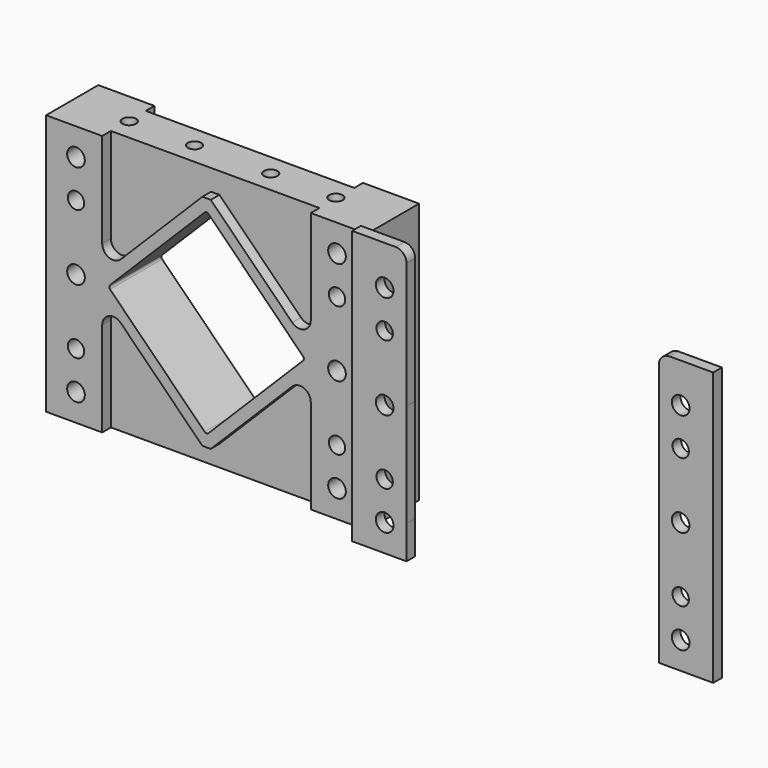
from build123d import *

# Parameters (mm, degrees)
F0_W      = 187.325
F0_H      = 152.4
F1_DEPTH  = 38.1
F3_D      = 9.5758
F4_DEPTH  = 6.35
F6_DEPTH  = 6.35
F8_D      = 7.9375
F8_DEPTH  = 22.225
F8_TIP    = 2.3846655818
F10_D     = 7.9375
F10_DEPTH = 22.225
F10_TIP   = 2.3846655818
F11_D     = 10.3124
F12_R     = 5.1562
F12_R_2   = 4.7879
F13_DEPTH = 6.35
F14_ANGLE = 180
F16_ANGLE = 180


# Not quite as in the source:
# - ends of sketch curves that miss each other by under 0.0002 mm in the source are joined


with BuildPart() as f1:
    # F0 (on Front) → F1 (new body)
    with BuildSketch(Plane.XZ):
        with Locations((17.3622183502, -12.1438738748)):
            Rectangle(F0_W, F0_H)
        with BuildLine():
            ThreePointArc((73.7470006338, -11.0550622269), (74.2119686187, -12.1775942421), (73.7470006338, -13.3001262572))
            Line((73.7470006338, -13.3001262572), (18.5184254892, -68.5287014018))
            ThreePointArc((18.5184254892, -68.5287014018), (17.3958934741, -68.9936693866), (16.273361459, -68.5287014018))
            Line((16.273361459, -68.5287014018), (-38.9552136856, -13.3001262572))
            ThreePointArc((-38.9552136856, -13.3001262572), (-39.4201816705, -12.1775942421), (-38.9552136856, -11.0550622269))
            Line((-38.9552136856, -11.0550622269), (16.273361459, 44.1735129177))
            ThreePointArc((16.273361459, 44.1735129177), (17.3958934741, 44.6384809025), (18.5184254892, 44.1735129177))
            Line((18.5184254892, 44.1735129177), (73.7470006338, -11.0550622269))
        make_face(mode=Mode.SUBTRACT)
    extrude(amount=F1_DEPTH)

    # F3 (through all)
    with Locations(Plane(origin=(0, 0, 0), x_dir=(1, 0, 0), z_dir=(0, 1, 0))):
        with Locations((-58.8377816498, -25.9561261252), (-58.8377816498, 50.2438738748), (93.5622183502, 50.2438738748), (93.5622183502, -25.9561261252)):
            Hole(F3_D / 2)

    # F2 (on face) → F4 (cut)
    with BuildSketch(Plane.XZ.offset(38.1)):
        with BuildLine():
            Line((-32.6721932196, 4.2082143602), (14.9574931524, 51.8379007322))
            Line((14.9574931524, 51.8379007322), (17.3622183502, 51.8379006441))
            Line((17.3622183502, 51.8379006441), (17.3622183502, 64.0561261252))
            Line((17.3622183502, 64.0561261252), (-43.5123212801, 64.0561261252))
            Line((-43.5123212801, 64.0561261252), (-43.5123212801, 8.6983424207))
            ThreePointArc((-43.5123212801, 8.6983424207), (-39.5923610756, 2.8317073892), (-32.6721932196, 4.2082143602))
        make_face()
        with BuildLine():
            Line((17.3622183502, 64.0561261252), (17.3622183502, 51.8379006441))
            Line((17.3622183502, 51.8379006441), (19.8342931524, 51.8379005536))
            Line((19.8342931524, 51.8379005536), (67.3966299199, 4.2755637861))
            ThreePointArc((67.3966299199, 4.2755637861), (74.316797776, 2.8990568152), (78.2367579805, 8.7656918466))
            Line((78.2367579805, 8.7656918466), (78.2367579805, 64.0561261252))
            Line((78.2367579805, 64.0561261252), (17.3622183502, 64.0561261252))
        make_face()
        with BuildLine():
            Line((19.8340516262, -76.1933300919), (17.3558846933, -76.1930850326))
            Line((17.3558846933, -76.1930850326), (17.354683134, -88.3438738748))
            Line((17.354683134, -88.3438738748), (78.2360174681, -88.3438738748))
            Line((78.2360174681, -88.3438738748), (78.2360174681, -33.1216203711))
            ThreePointArc((78.2360174681, -33.1216203711), (74.3160572637, -27.2549853396), (67.3958894076, -28.6314923106))
            Line((67.3958894076, -28.6314923106), (19.8340516262, -76.1933300919))
        make_face()
        with BuildLine():
            Line((17.354683134, -88.3438738748), (17.3558846933, -76.1930850326))
            Line((17.3558846933, -76.1930850326), (14.9572517743, -76.1928478381))
            Line((14.9572517743, -76.1928478381), (-32.6714527073, -28.5641433566))
            ThreePointArc((-32.6714527073, -28.5641433566), (-39.5916205633, -27.1876363857), (-43.5115807678, -33.0542714171))
            Line((-43.5115807678, -33.0542714171), (-43.5115807678, -88.3438738748))
            Line((-43.5115807678, -88.3438738748), (17.354683134, -88.3438738748))
        make_face()
    extrude(amount=-F4_DEPTH, mode=Mode.SUBTRACT)

    # F5 (on face) → F6 (cut)
    with BuildSketch(Plane.XZ):
        with BuildLine():
            Line((78.2333183502, -88.3438738748), (78.2333183502, -76.2026738748))
            Line((78.2333183502, -76.2026738748), (78.2333183502, -33.1243194891))
            ThreePointArc((78.2333183502, -33.1243194891), (74.3133581457, -27.2576844576), (67.3931902896, -28.6341914285))
            Line((67.3931902896, -28.6341914285), (19.8247078433, -76.2026738748))
            Line((19.8247078433, -76.2026738748), (14.967077811, -76.2026738748))
            Line((14.967077811, -76.2026738748), (-32.6687535893, -28.5668424746))
            ThreePointArc((-32.6687535893, -28.5668424746), (-39.5889214453, -27.1903355036), (-43.5088816498, -33.0569705351))
            Line((-43.5088816498, -33.0569705351), (-43.5088816498, -88.3438738748))
            Line((-43.5088816498, -88.3438738748), (78.2333183502, -88.3438738748))
        make_face()
        with BuildLine():
            Line((15.0345185454, 51.9149261252), (19.7572675809, 51.9149261252))
            Line((19.7572675809, 51.9149261252), (67.3931902896, 4.2790034164))
            ThreePointArc((67.3931902896, 4.2790034164), (74.3133581457, 2.9024964455), (78.2333183502, 8.7691314769))
            Line((78.2333183502, 8.7691314769), (78.2333183502, 64.0561261252))
            Line((78.2333183502, 64.0561261252), (-43.5088816498, 64.0561261252))
            Line((-43.5088816498, 64.0561261252), (-43.5088816498, 51.9149261252))
            Line((-43.5088816498, 51.9149261252), (-43.5088816498, 8.701782051))
            ThreePointArc((-43.5088816498, 8.701782051), (-39.5889214453, 2.8351470195), (-32.6687535893, 4.2116539905))
            Line((-32.6687535893, 4.2116539905), (15.0345185454, 51.9149261252))
        make_face()
    extrude(amount=F6_DEPTH, mode=Mode.SUBTRACT)

    # F8
    with Locations(Plane(origin=(0, 0, -88.3438738748), x_dir=(1, 0, 0), z_dir=(0, 0, -1))):
        with Locations((-42.9627816498, 19.05), (-4.8627816498, 19.05), (77.6872183502, 19.05), (39.5872183502, 19.05)):
            Hole(F8_D / 2, depth=F8_DEPTH)
            with Locations((0, 0, -(F8_DEPTH + F8_TIP / 2))):  # 118° drill point
                Cone(0, F8_D / 2, F8_TIP, mode=Mode.SUBTRACT)

    # F10
    with Locations(Plane.XY.offset(64.0561261252)):
        with Locations((-42.9627816498, -19.05), (-4.8627816498, -19.05), (39.5872183502, -19.05), (77.6872183502, -19.05)):
            Hole(F10_D / 2, depth=F10_DEPTH)
            with Locations((0, 0, -(F10_DEPTH + F10_TIP / 2))):  # 118° drill point
                Cone(0, F10_D / 2, F10_TIP, mode=Mode.SUBTRACT)

    # F11 (through all)
    with Locations(Plane(origin=(0, 0, 0), x_dir=(1, 0, 0), z_dir=(0, 1, 0))):
        with Locations((-58.8377816498, 72.4688738748), (-58.8377816498, 12.1438738748), (-58.8377816498, -48.1811261252), (93.5622183502, -48.1811261252), (93.5622183502, 12.1438738748), (93.5622183502, 72.4688738748)):
            Hole(F11_D / 2)


with BuildPart() as f13:
    # F12 (on face) → F13 (new body)
    with BuildSketch(Plane.XZ.offset(38.1)):
        Polygon((111.0247183502, 64.0561261252), (80.8068367085, 64.0561261252), (80.8068367085, 51.8378983214), (80.8068367085, -8.5778866934), (80.8068344967, -68.9936717082), (80.8068367085, -88.3438738748), (111.0247183502, -88.3438738748), align=None)
        with Locations((93.5622183502, -72.4688738748)):
            Circle(F12_R, mode=Mode.SUBTRACT)
        with Locations((93.5622183502, -50.2438738748)):
            Circle(F12_R_2, mode=Mode.SUBTRACT)
        with Locations((93.5622183502, -12.1438738748)):
            Circle(F12_R, mode=Mode.SUBTRACT)
        with Locations((93.5622183502, 25.9561261252)):
            Circle(F12_R_2, mode=Mode.SUBTRACT)
        with Locations((93.5622183502, 48.1811261252)):
            Circle(F12_R, mode=Mode.SUBTRACT)
        with BuildLine():
            Line((80.8068367085, 64.8507184755), (80.8068367085, 64.0561261252))
            Line((80.8068367085, 64.0561261252), (111.0247183502, 64.0561261252))
            Line((111.0247183502, 64.0561261252), (111.0247183502, -88.3438738748))
            Line((111.0247183502, -88.3438738748), (112.5568367085, -88.3438738748))
            Line((112.5568367085, -88.3438738748), (112.5568367085, -8.5778866934))
            Line((112.5568367085, -8.5778866934), (112.5568367085, 71.2007184755))
            Line((112.5568367085, 71.2007184755), (87.1568367085, 71.2007184755))
            ThreePointArc((87.1568367085, 71.2007184755), (82.666708648, 69.340846536), (80.8068367085, 64.8507184755))
        make_face()
    extrude(amount=F13_DEPTH)


with BuildPart() as f13_1:
    # F14: moved
    add(f13.part.rotate(Axis((112.5568367085, -44.45, -8.5715776997), (0, 0, 1)), F14_ANGLE))


with BuildPart() as f15_1:
    # F15: copy of F13
    add(f13_1.part.moved(Location((152.4, 0, 0))))


with BuildPart() as f15_1_1:
    # F16: moved
    add(f15_1.part.rotate(Axis((296.7068378145, -50.8, -78.6687727915), (1.143e-07, 0, 1)), F16_ANGLE))


solid = Compound([f1.part, f13_1.part, f15_1_1.part])
